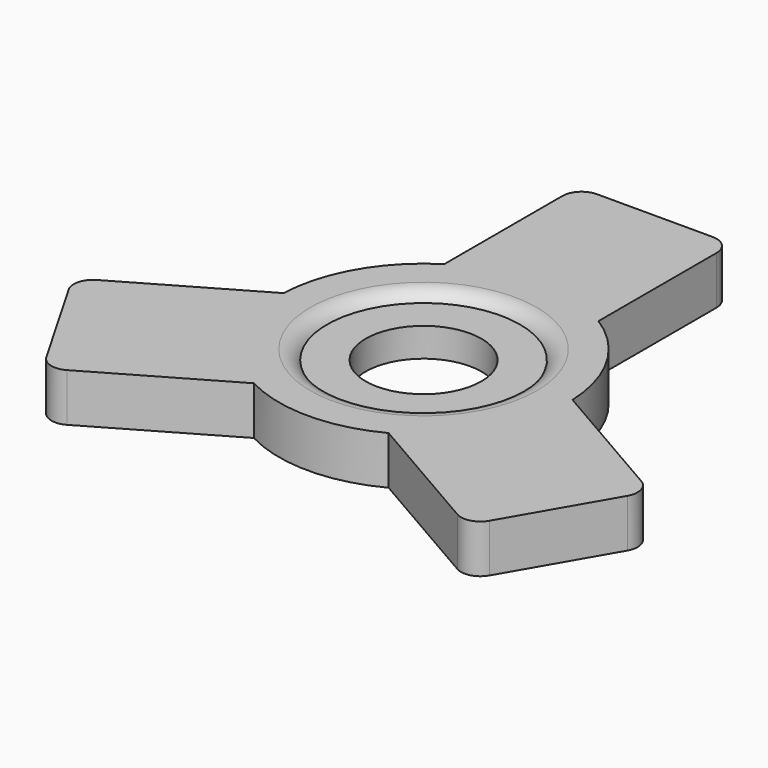
from build123d import *

# Parameters (mm, degrees)
F0_R        = 10
F1_DEPTH    = 2.5
F0_R_2      = 6
F2_DEPTH    = 1.5
F3_T1_DEPTH = 15


# Not quite as in the source:
# - a fillet or chamfer that OpenCascade refuses, or shapes differently, is made with other operations: its cross-section is extruded or revolved along the edge and cut away or added


with BuildPart() as f1:
    # F0 (on Top) → F1 (new body, symmetric)
    with BuildSketch(Plane.XY):
        with BuildLine():
            Line((25.9807621135, -15), (29.9807621135, -8.0717967697))
            Line((29.9807621135, -8.0717967697), (14.9886304879, 0.5839144601))
            ThreePointArc((14.9886304879, 0.5839144601), (12.9903810568, 7.5), (8, 12.6885775404))
            Line((8, 12.6885775404), (8, 30))
            Line((8, 30), (-8, 30))
            Line((-8, 30), (-8, 12.6885775404))
            ThreePointArc((-8, 12.6885775404), (-12.9903810568, 7.5), (-14.9886304879, 0.5839144601))
            Line((-14.9886304879, 0.5839144601), (-27.4269246123, -6.5973380009))
            Line((-27.4269246123, -6.5973380009), (-29.9807621135, -8.0717967697))
            Line((-29.9807621135, -8.0717967697), (-21.9807621135, -21.9282032303))
            Line((-21.9807621135, -21.9282032303), (-6.9886304879, -13.2724920005))
            ThreePointArc((-6.9886304879, -13.2724920005), (0, -15), (6.9886304879, -13.2724920005))
            Line((6.9886304879, -13.2724920005), (21.9807621135, -21.9282032303))
            Line((21.9807621135, -21.9282032303), (25.9807621135, -15))
        make_face()
        Circle(F0_R, mode=Mode.SUBTRACT)
    extrude(amount=F1_DEPTH, both=True)

    # F0 (on Top) → F2 (join, symmetric)
    with BuildSketch(Plane.XY):
        Circle(F0_R)
        Circle(F0_R_2, mode=Mode.SUBTRACT)
    extrude(amount=F2_DEPTH, both=True)

    # F3: fillet of radius 2 on 8 edges, made by hand

    # F3_s2 → F3_t1 (cut)
    with BuildSketch(Plane.XY.offset(-7.5)):
        with BuildLine():
            ThreePointArc((-28.9807621135, -9.8038475773), (-29.1805629585, -8.2862094871), (-28.248711306, -7.0717967697))
            Line((-28.248711306, -7.0717967697), (-29.9807621135, -8.0717967697))
            Line((-29.9807621135, -8.0717967697), (-28.9807621135, -9.8038475773))
        make_face()
        with BuildLine():
            ThreePointArc((-20.248711306, -20.9282032303), (-21.7663493962, -21.1280040753), (-22.9807621135, -20.1961524227))
            Line((-22.9807621135, -20.1961524227), (-21.9807621135, -21.9282032303))
            Line((-21.9807621135, -21.9282032303), (-20.248711306, -20.9282032303))
        make_face()
        with BuildLine():
            ThreePointArc((20.248711306, -20.9282032303), (21.7663493962, -21.1280040753), (22.9807621135, -20.1961524227))
            Line((22.9807621135, -20.1961524227), (21.9807621135, -21.9282032303))
            Line((21.9807621135, -21.9282032303), (20.248711306, -20.9282032303))
        make_face()
        with BuildLine():
            ThreePointArc((28.9807621135, -9.8038475773), (29.1805629585, -8.2862094871), (28.248711306, -7.0717967697))
            Line((28.248711306, -7.0717967697), (29.9807621135, -8.0717967697))
            Line((29.9807621135, -8.0717967697), (28.9807621135, -9.8038475773))
        make_face()
        with BuildLine():
            ThreePointArc((8, 28), (7.4142135624, 29.4142135624), (6, 30))
            Line((6, 30), (8, 30))
            Line((8, 30), (8, 28))
        make_face()
        with BuildLine():
            ThreePointArc((-6, 30), (-7.4142135624, 29.4142135624), (-8, 28))
            Line((-8, 28), (-8, 30))
            Line((-8, 30), (-6, 30))
        make_face()
    extrude(amount=F3_T1_DEPTH, mode=Mode.SUBTRACT)

    # F3_s3 → F3_t4 (revolve, cut)
    with BuildSketch(Plane.XZ):
        with BuildLine():
            ThreePointArc((11.7320508076, 2.5), (10.7320508076, 2.2320508076), (10, 1.5))
            Line((10, 1.5), (10, 2.5))
            Line((10, 2.5), (11.7320508076, 2.5))
        make_face()
    revolve(axis=Axis((0, 0, 2.5), (0, 0, 1)), mode=Mode.SUBTRACT)

    # F3_s5 → F3_t6 (revolve, cut)
    with BuildSketch(Plane.XZ):
        with BuildLine():
            ThreePointArc((11.7320508076, -2.5), (10.7320508076, -2.2320508076), (10, -1.5))
            Line((10, -1.5), (10, -2.5))
            Line((10, -2.5), (11.7320508076, -2.5))
        make_face()
    revolve(axis=Axis((0, 0, -2.5), (0, 0, 1)), mode=Mode.SUBTRACT)


solid = f1.part
